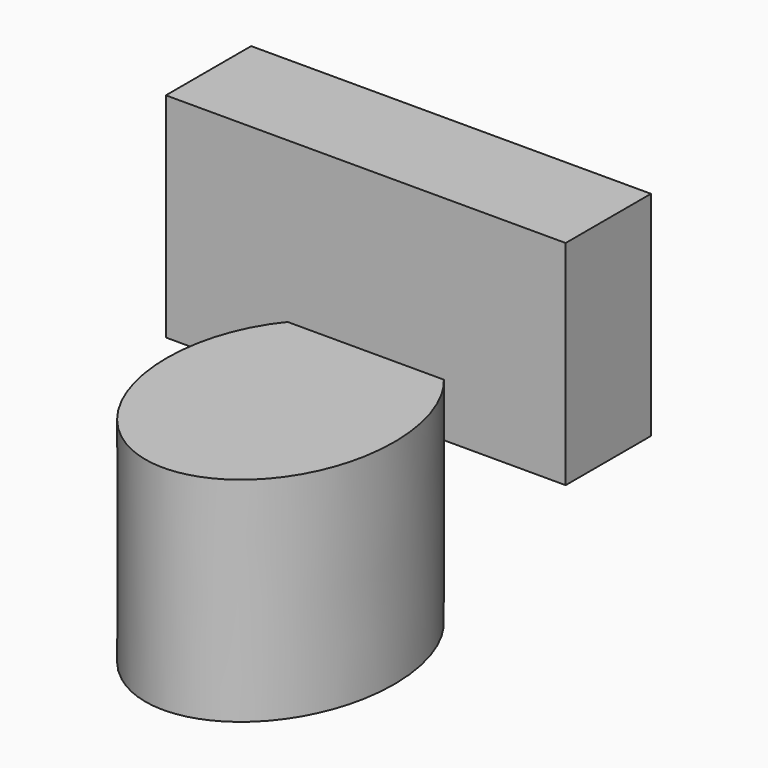
from build123d import *

# Parameters (mm, degrees)
F1_DEPTH = 406.4
F2_START = 304.8
F2_DEPTH = 406.4


# Not quite as in the source:
# - a feature names something its author has since deleted; it is built from what else it names


with BuildPart() as f1:
    # F0 (on Top) → F1 (new body)
    with BuildSketch(Plane.XY):
        with BuildLine():
            Line((19.4174144417, -203.2), (145.9747472738, -203.2))
            add(Edge.make_bspline(
                [(145.9747472738, -203.2), (83.2877280017, -127), (-2.9069234974, -127)],
                knots=[5.5267289225, 5.5267289225, 5.5267289225, 6.2831853072, 6.2831853072, 6.2831853072], degree=2, weights=[1, 0.9293203773, 1]))
            add(Edge.make_bspline(
                [(-2.9069234974, -127), (-89.1015749965, -127), (-151.7885942685, -203.2)],
                knots=[0, 0, 0, 0.7564563847, 0.7564563847, 0.7564563847], degree=2, weights=[1, 0.9293203773, 1]))
            Line((-151.7885942685, -203.2), (19.4174144417, -203.2))
        make_face()
        with BuildLine():
            add(Edge.make_bspline(
                [(-151.7885942685, -203.2), (-548.8063829917, -685.8), (-2.9069234974, -685.8), (542.992535997, -685.8), (145.9747472738, -203.2)],
                knots=[0.7564563847, 0.7564563847, 0.7564563847, 3.1415926536, 3.1415926536, 5.5267289225, 5.5267289225, 5.5267289225], degree=2, weights=[1, 0.3692744729, 1, 0.3692744729, 1]))
            Line((145.9747472738, -203.2), (19.4174144417, -203.2))
            Line((19.4174144417, -203.2), (-151.7885942685, -203.2))
        make_face()
    extrude(amount=F1_DEPTH)

    # F0 (on Top) → F2 (join)
    with BuildSketch(Plane.XY.offset(F2_START)):
        with BuildLine():
            Line((378.0930765026, 0), (-383.9069234974, 0))
            Line((-383.9069234974, 0), (-383.9069234974, -203.2))
            Line((-383.9069234974, -203.2), (-286.6143286228, -203.2))
            Line((-286.6143286228, -203.2), (-151.7885942685, -203.2))
            add(Edge.make_bspline(
                [(-2.9069234974, -127), (-89.1015749965, -127), (-151.7885942685, -203.2)],
                knots=[0, 0, 0, 0.7564563847, 0.7564563847, 0.7564563847], degree=2, weights=[1, 0.9293203773, 1]))
            add(Edge.make_bspline(
                [(145.9747472738, -203.2), (83.2877280017, -127), (-2.9069234974, -127)],
                knots=[5.5267289225, 5.5267289225, 5.5267289225, 6.2831853072, 6.2831853072, 6.2831853072], degree=2, weights=[1, 0.9293203773, 1]))
            Line((145.9747472738, -203.2), (378.0930765026, -203.2))
            Line((378.0930765026, -203.2), (378.0930765026, 0))
        make_face()
        with BuildLine():
            Line((19.4174144417, -203.2), (145.9747472738, -203.2))
            add(Edge.make_bspline(
                [(145.9747472738, -203.2), (83.2877280017, -127), (-2.9069234974, -127)],
                knots=[5.5267289225, 5.5267289225, 5.5267289225, 6.2831853072, 6.2831853072, 6.2831853072], degree=2, weights=[1, 0.9293203773, 1]))
            add(Edge.make_bspline(
                [(-2.9069234974, -127), (-89.1015749965, -127), (-151.7885942685, -203.2)],
                knots=[0, 0, 0, 0.7564563847, 0.7564563847, 0.7564563847], degree=2, weights=[1, 0.9293203773, 1]))
            Line((-151.7885942685, -203.2), (19.4174144417, -203.2))
        make_face()
    extrude(amount=F2_DEPTH)


solid = f1.part
